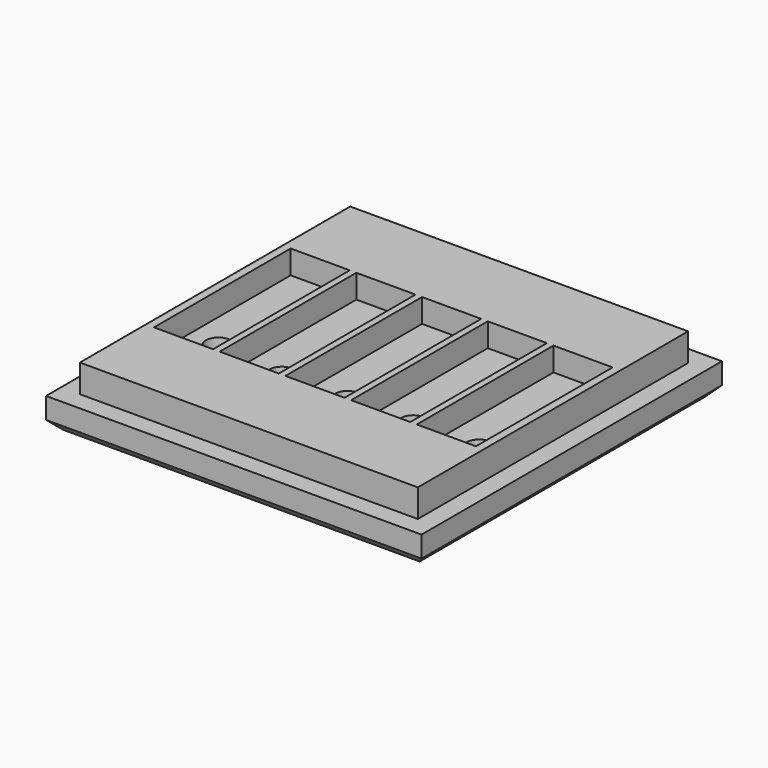
from build123d import *

# Parameters (mm, degrees)
F0_W      = 50.8
F0_H      = 50.8
F1_DEPTH  = 4.13
F3_W      = 45.72
F3_H      = 45.72
F4_DEPTH  = 3.77
F5_W      = 8
F5_H      = 23.114
F6_DEPTH  = 3.2
F7_R      = 1.715
F8_DEPTH  = 25.4
F9_SIZE   = 1.27
F10_R     = 1.694213851
F11_DEPTH = 25.4


# Not quite as in the source:
# - a feature names something its author has since deleted; it is built from what else it names


with BuildPart() as f1:
    # F0 (on Top) → F1 (new body)
    with BuildSketch(Plane.XY):
        with Locations((13.0843408406, 14.7212249442)):
            Rectangle(F0_W, F0_H)
    extrude(amount=F1_DEPTH)

    # F3 (on face) → F4 (join)
    with BuildSketch(Plane.XY.offset(4.13)):
        with Locations((13.0843408406, 14.7212249442)):
            Rectangle(F3_W, F3_H)
    extrude(amount=F4_DEPTH)

    # F5 (on face) → F6 (cut)
    with BuildSketch(Plane.XY.offset(7.9)):
        with Locations((4.2001288666, 14.5942249442)):
            Rectangle(F5_W, F5_H)
        with Locations((13.0901288666, 14.5942249442)):
            Rectangle(F5_W, F5_H)
        with Locations((21.9801288666, 14.5942249442)):
            Rectangle(F5_W, F5_H)
        with Locations((30.8701288666, 14.5942249442)):
            Rectangle(F5_W, F5_H)
        with Locations((-4.6898711334, 14.5942249442)):
            Rectangle(F5_W, F5_H)
    extrude(amount=-F6_DEPTH, mode=Mode.SUBTRACT)

    # F7 (on face) → F8 (cut)
    with BuildSketch(Plane.XY.offset(4.7)):
        with Locations((-4.6898711334, 8.9522249442)):
            Circle(F7_R)
    extrude(amount=-F8_DEPTH, mode=Mode.SUBTRACT)

    # F9
    f9_edges = [f1.edges().sort_by_distance(p)[0] for p in [
        (13.084341, -10.678775, 0),
        (13.084341, 40.121225, 0),
        (-12.315659, 14.721225, 0),
        (38.484341, 14.721225, 0),
    ]]
    chamfer(f9_edges, length=F9_SIZE)

    # F10 (on face) → F11 (cut)
    with BuildSketch(Plane.XY.offset(4.7)):
        with Locations((4.7001288666, 7.9312249442)):
            Circle(F10_R)
        with Locations((13.5901288666, 7.9312249442)):
            Circle(F10_R)
        with Locations((22.4801288666, 7.9312249442)):
            Circle(F10_R)
        with Locations((31.3701288666, 7.9394249442)):
            Circle(F10_R)
    extrude(amount=-F11_DEPTH, mode=Mode.SUBTRACT)


solid = f1.part
